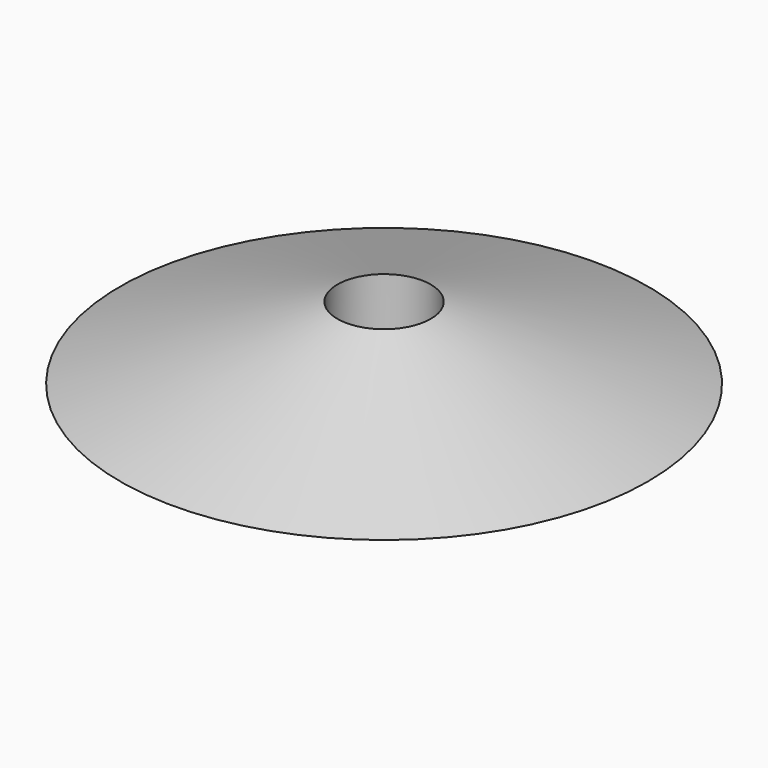
from build123d import *

# Parameters (mm, degrees)
F2_R     = 2.65
F3_DEPTH = 44


# Not quite as in the source:
# - an extrude ends at something that could not be found from the text; its depth is read off the source's solid


with BuildPart() as f1:
    # F0 (on Front) → F1 (revolve)
    with BuildSketch(Plane.XZ):
        Polygon((0, 5), (0, 0), (15, 0), align=None)
    revolve(axis=Axis((0, 0, 2.5), (0, 0, -1)))

    # F2 (on face) → F3 (cut, through all)
    with BuildSketch(Plane(origin=(0, 0, 0), x_dir=(1, 0, 0), z_dir=(0, 0, -1))):
        Circle(F2_R)
    extrude(amount=-F3_DEPTH, mode=Mode.SUBTRACT)


solid = f1.part
